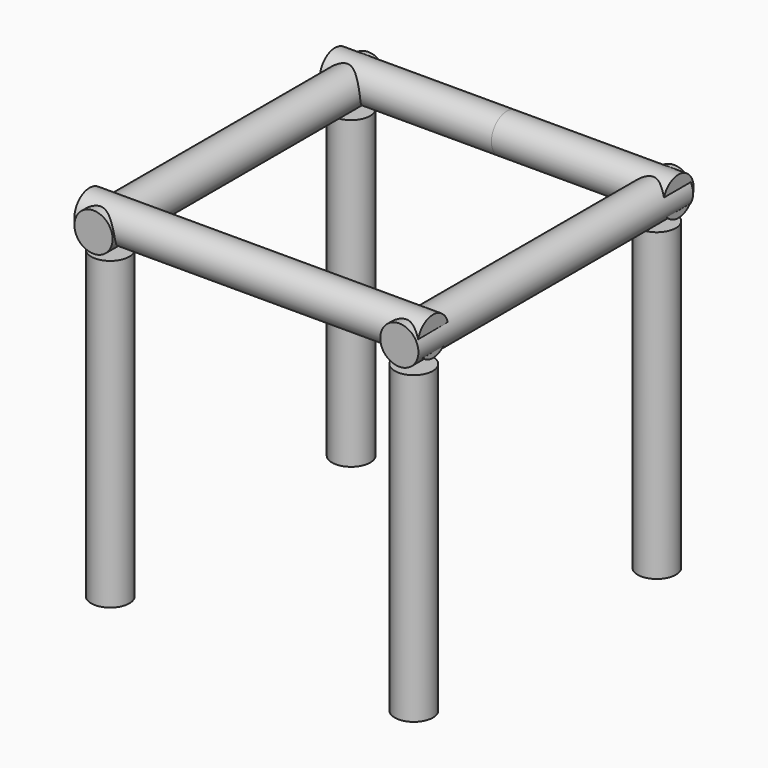
from build123d import *

# Parameters (mm, degrees)
F0_R     = 6.35
F1_DEPTH = 101.6
F2_R     = 6.35
F3_DEPTH = 57.15
F4_R     = 6.35
F5_DEPTH = 57.15


with BuildPart() as f1:
    # F0 (on Top) → F1 (new body)
    with BuildSketch(Plane.XY):
        with Locations((51.6017824411, -51.1305369437)):
            Circle(F0_R)
    extrude(amount=F1_DEPTH)


with BuildPart() as f1b:
    # F0 (on Top) → F1, piece 2 (new body)
    with BuildSketch(Plane.XY):
        with Locations((-50.1880459487, -50.1880384982)):
            Circle(F0_R)
    extrude(amount=F1_DEPTH)


with BuildPart() as f1c:
    # F0 (on Top) → F1, piece 3 (new body)
    with BuildSketch(Plane.XY):
        with Locations((-50.8, 50.8)):
            Circle(F0_R)
    extrude(amount=F1_DEPTH)


with BuildPart() as f1d:
    # F0 (on Top) → F1, piece 4 (new body)
    with BuildSketch(Plane.XY):
        with Locations((50.6592802703, 51.130540669)):
            Circle(F0_R)
    extrude(amount=F1_DEPTH)


with BuildPart() as f3:
    # F2 (on Front) → F3 (new body, symmetric)
    with BuildSketch(Plane.XZ):
        with Locations((-50.1880459487, 109.5654368401)):
            Circle(F2_R)
    extrude(amount=F3_DEPTH, both=True)


with BuildPart() as f3b:
    # F2 (on Front) → F3, piece 2 (new body, symmetric)
    with BuildSketch(Plane.XZ):
        with Locations((51.6017861664, 109.5654368401)):
            Circle(F2_R)
    extrude(amount=F3_DEPTH, both=True)

    # F4 (on Right) → F5 (join, symmetric)
    with BuildSketch(Plane.YZ):
        with Locations((52.0190373063, 110.5906814337)):
            Circle(F4_R)
        with Locations((-50.0834435225, 111.0794693232)):
            Circle(F4_R)
    extrude(amount=F5_DEPTH, both=True)


solid = Compound([f1.part, f1b.part, f1c.part, f1d.part, f3.part, f3b.part])
